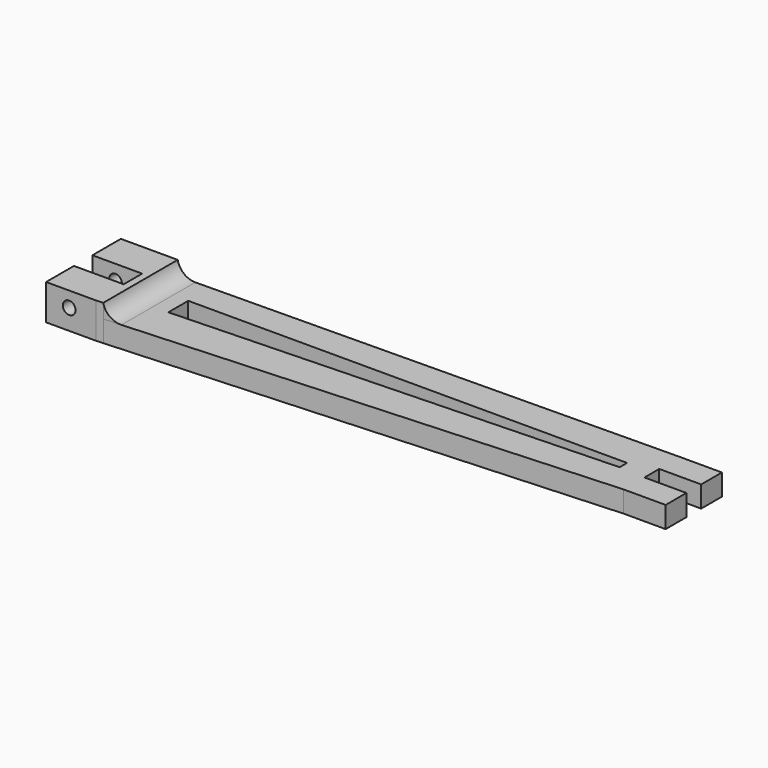
from build123d import *

# Parameters (mm, degrees)
F0_W        = 5.8
F0_H        = 7.3
F0_W_2      = 14
F0_H_2      = 9.8
F0_W_3      = 6
F1_DEPTH    = 6
F2_DEPTH    = 10
F3_R        = 1.8
F4_DEPTH    = 46
F5_T4_DEPTH = 50.6794044701


# Not quite as in the source:
# - a fillet or chamfer that OpenCascade refuses, or shapes differently, is made with other operations: its cross-section is extruded or revolved along the edge and cut away or added


with BuildPart() as f1:
    # F0 (on Top) → F1 (new body)
    with BuildSketch(Plane.XY):
        with Locations((49.0534804702, 31.8385251075)):
            Rectangle(F0_W, F0_H)
        with Locations((49.0534804702, 19.3385251075)):
            Rectangle(F0_W, F0_H)
        with Locations((-108.8465195298, 12.3885251075)):
            Rectangle(F0_W_2, F0_H_2)
        with Locations((43.1534804702, 31.8385251075)):
            Rectangle(F0_W_3, F0_H)
        with Locations((43.1534804702, 19.3385251075)):
            Rectangle(F0_W_3, F0_H)
        Polygon((-99.8465195298, 7.6040180652), (-99.8465195298, 33.7885251075), (-115.8465195298, 33.7885251075), (-115.8465195298, 31.2885251075), (-115.8465195298, 23.7885251075), (-101.8465195298, 23.7885251075), (-101.8465195298, 17.2885251075), (-101.8465195298, 7.4885251075), align=None)
        Polygon((40.1534804702, 28.1885251075), (40.1534804702, 35.4885251075), (-99.8465195298, 33.7885251075), (-99.8465195298, 7.6040180652), (40.1534804702, 15.6885251075), (40.1534804702, 22.9885251075), align=None)
        Polygon((-90.6591936946, 19.0157179874), (-90.6591936946, 26.0108020157), (32.8437909484, 26.0108020157), (32.8437909484, 23.3903356981), align=None, mode=Mode.SUBTRACT)
    extrude(amount=F1_DEPTH)

    # F0 (on Top) → F2 (join)
    with BuildSketch(Plane.XY):
        Polygon((-99.8465195298, 7.6040180652), (-99.8465195298, 33.7885251075), (-115.8465195298, 33.7885251075), (-115.8465195298, 31.2885251075), (-115.8465195298, 23.7885251075), (-101.8465195298, 23.7885251075), (-101.8465195298, 17.2885251075), (-101.8465195298, 7.4885251075), align=None)
        with Locations((-108.8465195298, 12.3885251075)):
            Rectangle(F0_W_2, F0_H_2)
    extrude(amount=F2_DEPTH)

    # F3 (on Front) → F4 (cut)
    with BuildSketch(Plane.XZ):
        with Locations((-109.3465195298, 5.7222666219)):
            Circle(F3_R)
    extrude(amount=-F4_DEPTH, mode=Mode.SUBTRACT)

    # F5: fillet of radius 5 on 1 edges, made by hand


with BuildPart() as f5_tool2:
    # F5_s3 → F5_t4 (new body)
    with BuildSketch(Plane.XZ.offset(-46.0359738214)):
        with BuildLine():
            ThreePointArc((-94.9475400442, 6), (-98.1098177044, 7.1270166538), (-99.8465195298, 10))
            Line((-99.8465195298, 10), (-99.8465195298, 6))
            Line((-99.8465195298, 6), (-94.9475400442, 6))
        make_face()
    extrude(amount=F5_T4_DEPTH)

    split(bisect_by=Plane(origin=(-0.4249488426, 34.9957870373, 0), x_dir=(0, 0, 1), z_dir=(0.012141962, -0.9999262837, 0)), keep=Keep.TOP)

    split(bisect_by=Plane(origin=(-0.7694930518, 13.3253674816, 0), x_dir=(0, 0, 1), z_dir=(-0.0576504367, 0.9983368305, 0)), keep=Keep.TOP)


with BuildPart() as f1_1:
    add(f1.part)

    # F5_t1: union F5_tool2
    add(f5_tool2.part)


solid = f1_1.part
